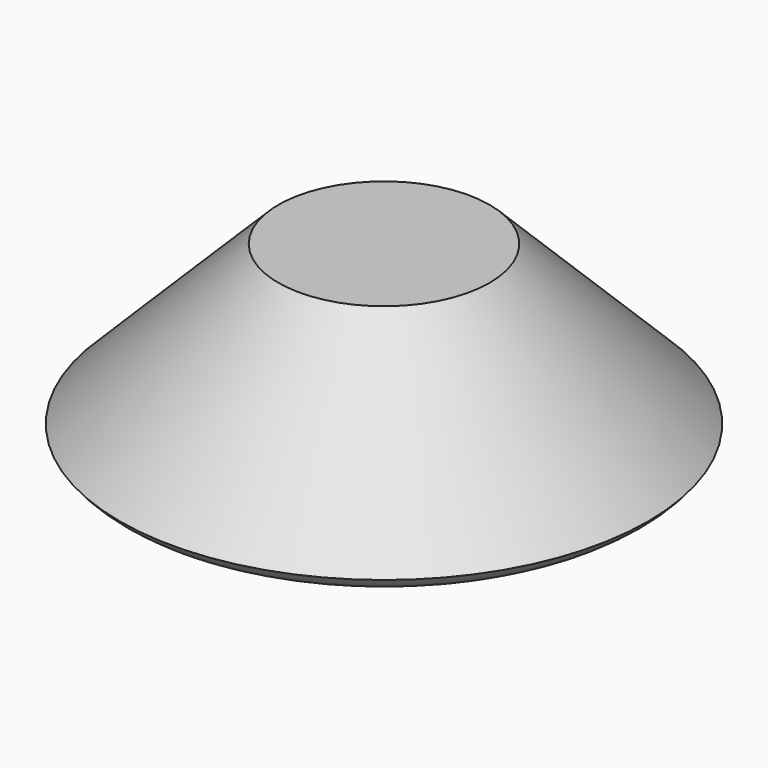
from build123d import *

# Parameters (mm, degrees)
F0_R     = 25
F1_DEPTH = 17
F2_SIZE  = 15


# Not quite as in the source:
# - a fillet or chamfer that OpenCascade refuses, or shapes differently, is made with other operations: its cross-section is extruded or revolved along the edge and cut away or added


with BuildPart() as f1:
    # F0 (on Top) → F1 (new body)
    with BuildSketch(Plane.XY):
        with Locations((-14.6842114627, 6.9868424907)):
            Circle(F0_R)
    extrude(amount=F1_DEPTH)

    # F2
    f2_edges = [f1.edges().sort_by_distance(p)[0] for p in [
        (-39.684211, 6.986842, 17),
    ]]
    chamfer(f2_edges, length=F2_SIZE)

    # F3: fillet of radius 5 on 1 edges, made by hand

    # F3_s1 → F3_t2 (revolve, cut)
    with BuildSketch(Plane.XZ.offset(-6.9868424907)):
        with BuildLine():
            ThreePointArc((10.3157885373, 2), (8.5518565148, 0.527864045), (6.3157885373, 0))
            Line((6.3157885373, 0), (10.3157885373, 0))
            Line((10.3157885373, 0), (10.3157885373, 2))
        make_face()
    revolve(axis=Axis((-14.6842114627, 6.9868424907, 0), (0, 0, 1)), mode=Mode.SUBTRACT)


solid = f1.part
